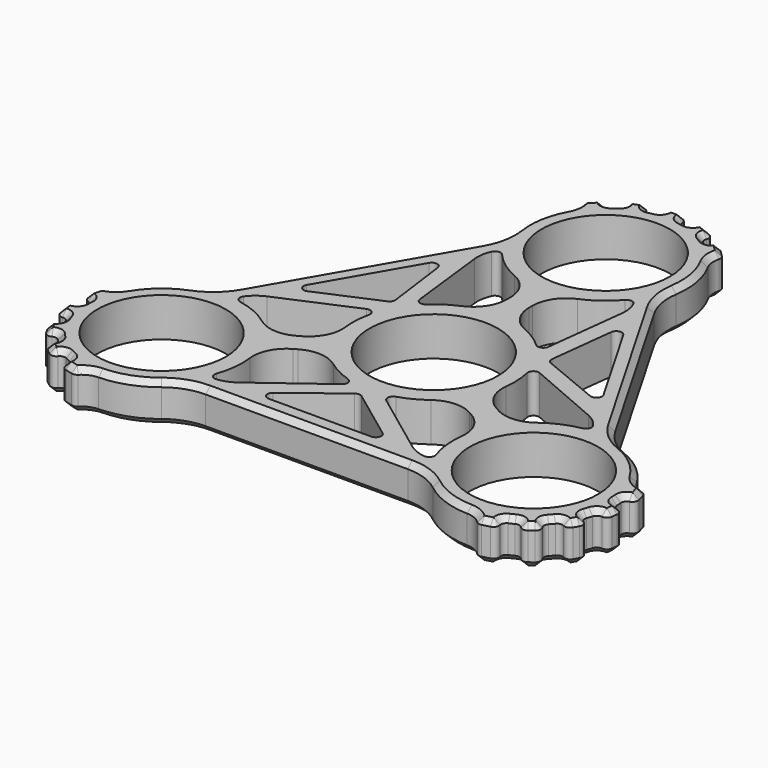
from build123d import *

# Parameters (mm, degrees)
F0_R        = 11.5
F1_DEPTH    = 7
F2_R        = 6
F3_R        = 1
F4_R        = 10
F5_T1_DEPTH = 7
F6_R        = 1
F7_R        = 1
F8_SIZE     = 0.9999


# Not quite as in the source:
# - a fillet or chamfer that OpenCascade refuses, or shapes differently, is made with other operations: its cross-section is extruded or revolved along the edge and cut away or added
# - a fillet or chamfer is up to 0.001 mm smaller than in the source, because OpenCascade refuses the exact size


with BuildPart() as f1:
    # F0 (on Top) → F1 (new body)
    with BuildSketch(Plane.XY):
        with BuildLine():
            Line((-12.5511453661, 48.9298250225), (-11.258699199, 47.6373788554))
            ThreePointArc((-11.258699199, 47.6373788554), (-14.3149781336, 40.8089826842), (-13.5606585567, 33.3659431724))
            Line((-13.5606585567, 33.3659431724), (-35.6760836869, -4.9390967841))
            ThreePointArc((-35.6760836869, -4.9390967841), (-42.4991047739, -8.0073566238), (-46.884529858, -14.0683699078))
            Line((-46.884529858, -14.0683699078), (-48.6500441552, -13.5953017777))
            Line((-48.6500441552, -13.5953017777), (-49.4265012906, -16.4930792565))
            Line((-49.4265012906, -16.4930792565), (-47.6609869933, -16.9661473867))
            ThreePointArc((-47.6609869933, -16.9661473867), (-47.8109324327, -18.3016546262), (-47.8365884719, -19.6453082233))
            Line((-47.8365884719, -19.6453082233), (-49.6487463314, -19.8838833315))
            Line((-49.6487463314, -19.8838833315), (-49.2571677547, -22.8582179156))
            Line((-49.2571677547, -22.8582179156), (-47.4450098953, -22.6196428074))
            ThreePointArc((-47.4450098953, -22.6196428074), (-47.0724649234, -23.9108722469), (-46.5819740425, -25.1620644453))
            Line((-46.5819740425, -25.1620644453), (-48.1648908572, -26.0759618943))
            Line((-48.1648908572, -26.0759618943), (-46.6648908572, -28.6740381057))
            Line((-46.6648908572, -28.6740381057), (-45.0819740425, -27.7601406566))
            ThreePointArc((-45.0819740425, -27.7601406566), (-44.2436552541, -28.810514319), (-43.3116902434, -29.7787624484))
            Line((-43.3116902434, -29.7787624484), (-44.4243812775, -31.2288496362))
            Line((-44.4243812775, -31.2288496362), (-42.0443212567, -33.0551339232))
            Line((-42.0443212567, -33.0551339232), (-40.9316302225, -31.6050467354))
            ThreePointArc((-40.9316302225, -31.6050467354), (-39.7551640539, -32.2546547522), (-38.5236081379, -32.7925518123))
            Line((-38.5236081379, -32.7925518123), (-38.9966762681, -34.5580661095))
            Line((-38.9966762681, -34.5580661095), (-36.0988987892, -35.3345232449))
            Line((-36.0988987892, -35.3345232449), (-35.625830659, -33.5690089476))
            ThreePointArc((-35.625830659, -33.5690089476), (-28.1841266403, -32.8016260604), (-22.1154251302, -28.4268463883))
            Line((-22.1154251302, -28.4268463883), (22.1154251302, -28.4268463883))
            ThreePointArc((22.1154251302, -28.4268463883), (28.1841266403, -32.8016260604), (35.625830659, -33.5690089476))
            Line((35.625830659, -33.5690089476), (36.0988987892, -35.3345232449))
            Line((36.0988987892, -35.3345232449), (38.9966762681, -34.5580661095))
            Line((38.9966762681, -34.5580661095), (38.5236081379, -32.7925518123))
            ThreePointArc((38.5236081379, -32.7925518123), (39.7551640539, -32.2546547522), (40.9316302225, -31.6050467354))
            Line((40.9316302225, -31.6050467354), (42.0443212567, -33.0551339232))
            Line((42.0443212567, -33.0551339232), (44.4243812775, -31.2288496362))
            Line((44.4243812775, -31.2288496362), (43.3116902434, -29.7787624484))
            ThreePointArc((43.3116902434, -29.7787624484), (44.2436552541, -28.810514319), (45.0819740425, -27.7601406566))
            Line((45.0819740425, -27.7601406566), (46.6648908572, -28.6740381057))
            Line((46.6648908572, -28.6740381057), (48.1648908572, -26.0759618943))
            Line((48.1648908572, -26.0759618943), (46.5819740425, -25.1620644453))
            ThreePointArc((46.5819740425, -25.1620644453), (47.0724649234, -23.9108722469), (47.4450098953, -22.6196428074))
            Line((47.4450098953, -22.6196428074), (49.2571677547, -22.8582179156))
            Line((49.2571677547, -22.8582179156), (49.6487463314, -19.8838833315))
            Line((49.6487463314, -19.8838833315), (47.8365884719, -19.6453082233))
            ThreePointArc((47.8365884719, -19.6453082233), (47.8109324327, -18.3016546262), (47.6609869933, -16.9661473867))
            Line((47.6609869933, -16.9661473867), (49.4265012906, -16.4930792565))
            Line((49.4265012906, -16.4930792565), (48.6500441552, -13.5953017777))
            Line((48.6500441552, -13.5953017777), (46.884529858, -14.0683699078))
            ThreePointArc((46.884529858, -14.0683699078), (42.4991047739, -8.0073566238), (35.6760836869, -4.9390967841))
            Line((35.6760836869, -4.9390967841), (13.5606585567, 33.3659431724))
            ThreePointArc((13.5606585567, 33.3659431724), (14.3149781336, 40.8089826842), (11.258699199, 47.6373788554))
            Line((11.258699199, 47.6373788554), (12.5511453661, 48.9298250225))
            Line((12.5511453661, 48.9298250225), (10.4298250225, 51.0511453661))
            Line((10.4298250225, 51.0511453661), (9.1373788554, 49.758699199))
            ThreePointArc((9.1373788554, 49.758699199), (8.0557683788, 50.5563093784), (6.9049582494, 51.2503549587))
            Line((6.9049582494, 51.2503549587), (7.6044250747, 52.9390172548))
            Line((7.6044250747, 52.9390172548), (4.8327864772, 54.0870675519))
            Line((4.8327864772, 54.0870675519), (4.1333196519, 52.3984052558))
            ThreePointArc((4.1333196519, 52.3984052558), (2.8288096692, 52.7213865658), (1.5, 52.9222051019))
            Line((1.5, 52.9222051019), (1.5, 54.75))
            Line((1.5, 54.75), (-1.5, 54.75))
            Line((-1.5, 54.75), (-1.5, 52.9222051019))
            ThreePointArc((-1.5, 52.9222051019), (-2.8288096692, 52.7213865658), (-4.1333196519, 52.3984052558))
            Line((-4.1333196519, 52.3984052558), (-4.8327864772, 54.0870675519))
            Line((-4.8327864772, 54.0870675519), (-7.6044250747, 52.9390172548))
            Line((-7.6044250747, 52.9390172548), (-6.9049582494, 51.2503549587))
            ThreePointArc((-6.9049582494, 51.2503549587), (-8.0557683788, 50.5563093784), (-9.1373788554, 49.758699199))
            Line((-9.1373788554, 49.758699199), (-10.4298250225, 51.0511453661))
            Line((-10.4298250225, 51.0511453661), (-12.5511453661, 48.9298250225))
        make_face()
        with Locations((-33.3419780457, -19.25)):
            Circle(F0_R, mode=Mode.SUBTRACT)
        Polygon((-12.1679823131, -25.4268463883), (-0.1996260557, -16.2213186658), (12.1679823131, -25.4268463883), align=None, mode=Mode.SUBTRACT)
        with BuildLine():
            Line((-19.9046350819, -13.8013474994), (-11.4373429638, -8.9127541157))
            ThreePointArc((-11.4373429638, -8.9127541157), (-7.3686040003, -12.4881413784), (-2.2716589425, -14.3209484899))
            Line((-2.2716589425, -14.3209484899), (-17.1924109007, -25.4268463883))
            Line((-17.1924109007, -25.4268463883), (-20.2234198667, -25.4268463883))
            ThreePointArc((-20.2234198667, -25.4268463883), (-18.8474263976, -19.6474575692), (-19.9046350819, -13.8013474994))
        make_face(mode=Mode.SUBTRACT)
        with BuildLine():
            ThreePointArc((-13.5381346697, 5.193159892), (-14.4993496799, -0.1373275655), (-13.4373429638, -5.4486525006))
            Line((-13.4373429638, -5.4486525006), (-21.9046350819, -10.3372458843))
            ThreePointArc((-21.9046350819, -10.3372458843), (-26.4389105735, -6.4986212717), (-32.1320048438, -4.8005721618))
            Line((-32.1320048438, -4.8005721618), (-30.6165003608, -2.1756413982))
            Line((-30.6165003608, -2.1756413982), (-13.5381346697, 5.193159892))
        make_face(mode=Mode.SUBTRACT)
        with BuildLine():
            ThreePointArc((2.2716589425, -14.3209484899), (7.3686040003, -12.4881413784), (11.4373429638, -8.9127541157))
            Line((11.4373429638, -8.9127541157), (19.9046350819, -13.8013474994))
            ThreePointArc((19.9046350819, -13.8013474994), (18.8474263976, -19.6474575692), (20.2234198667, -25.4268463883))
            Line((20.2234198667, -25.4268463883), (17.1924109007, -25.4268463883))
            Line((17.1924109007, -25.4268463883), (2.2716589425, -14.3209484899))
        make_face(mode=Mode.SUBTRACT)
        with Locations((33.3419780457, -19.25)):
            Circle(F0_R, mode=Mode.SUBTRACT)
        with BuildLine():
            Line((21.9046350819, -10.3372458843), (13.4373429638, -5.4486525006))
            ThreePointArc((13.4373429638, -5.4486525006), (14.4993496799, -0.1373275655), (13.5381346697, 5.193159892))
            Line((13.5381346697, 5.193159892), (30.6165003608, -2.1756413982))
            Line((30.6165003608, -2.1756413982), (32.1320048438, -4.8005721618))
            ThreePointArc((32.1320048438, -4.8005721618), (26.4389105735, -6.4986212717), (21.9046350819, -10.3372458843))
        make_face(mode=Mode.SUBTRACT)
        Circle(F0_R, mode=Mode.SUBTRACT)
        Polygon((-15.9363037538, 23.2512049902), (-13.9482610196, 8.2835405684), (-28.104286067, 2.1756413982), align=None, mode=Mode.SUBTRACT)
        with BuildLine():
            Line((-2, 24.1385933837), (-2, 14.3614066163))
            ThreePointArc((-2, 14.3614066163), (-7.1307456795, 12.6254689439), (-11.2664757273, 9.1277885979))
            Line((-11.2664757273, 9.1277885979), (-13.42408946, 27.6024877865))
            Line((-13.42408946, 27.6024877865), (-11.9085849771, 30.2274185502))
            ThreePointArc((-11.9085849771, 30.2274185502), (-7.5914841759, 26.1460788408), (-2, 24.1385933837))
        make_face(mode=Mode.SUBTRACT)
        with BuildLine():
            ThreePointArc((11.2664757273, 9.1277885979), (7.1307456795, 12.6254689439), (2, 14.3614066163))
            Line((2, 14.3614066163), (2, 24.1385933837))
            ThreePointArc((2, 24.1385933837), (7.5914841759, 26.1460788408), (11.9085849771, 30.2274185502))
            Line((11.9085849771, 30.2274185502), (13.42408946, 27.6024877865))
            Line((13.42408946, 27.6024877865), (11.2664757273, 9.1277885979))
        make_face(mode=Mode.SUBTRACT)
        Polygon((28.104286067, 2.1756413982), (14.1478870753, 7.9377780974), (15.9363037538, 23.2512049902), align=None, mode=Mode.SUBTRACT)
        with Locations((0, 38.5)):
            Circle(F0_R, mode=Mode.SUBTRACT)
    extrude(amount=F1_DEPTH)

    # F2
    f2_edges = [f1.edges().sort_by_distance(p)[0] for p in [
        (-2, 14.361407, 3.5),
        (2, 14.361407, 3.5),
        (2, 24.138593, 3.5),
        (-2, 24.138593, 3.5),
        (-13.437343, -5.448653, 3.5),
        (19.904635, -13.801347, 3.5),
        (-19.904635, -13.801347, 3.5),
        (-11.437343, -8.912754, 3.5),
        (-21.904635, -10.337246, 3.5),
        (21.904635, -10.337246, 3.5),
        (11.437343, -8.912754, 3.5),
        (13.437343, -5.448653, 3.5),
        (-30.6165, -2.175641, 3.5),
        (-17.192411, -25.426846, 3.5),
        (17.192411, -25.426846, 3.5),
        (13.424089, 27.602488, 3.5),
        (30.6165, -2.175641, 3.5),
        (-13.424089, 27.602488, 3.5),
    ]]
    fillet(f2_edges, radius=F2_R)

    # F3
    f3_edges = [f1.edges().sort_by_distance(p)[0] for p in [
        (-11.266476, 9.127789, 3.5),
        (-13.538135, 5.19316, 3.5),
        (-2.271659, -14.320948, 3.5),
        (2.271659, -14.320948, 3.5),
        (13.538135, 5.19316, 3.5),
        (11.266476, 9.127789, 3.5),
        (32.132005, -4.800572, 3.5),
        (20.22342, -25.426846, 3.5),
        (-20.22342, -25.426846, 3.5),
        (-32.132005, -4.800572, 3.5),
        (11.908585, 30.227419, 3.5),
        (-11.908585, 30.227419, 3.5),
        (-15.936304, 23.251205, 3.5),
        (-28.104286, 2.175641, 3.5),
        (28.104286, 2.175641, 3.5),
        (15.936304, 23.251205, 3.5),
        (12.167982, -25.426846, 3.5),
        (-12.167982, -25.426846, 3.5),
        (-13.948261, 8.283541, 3.5),
        (-0.199626, -16.221319, 3.5),
        (14.147887, 7.937778, 3.5),
    ]]
    fillet(f3_edges, radius=F3_R)

    # F4
    f4_edges = [f1.edges().sort_by_distance(p)[0] for p in [
        (-13.560659, 33.365943, 3.5),
        (13.560659, 33.365943, 3.5),
        (-35.676084, -4.939097, 3.5),
        (-22.115425, -28.426846, 3.5),
        (22.115425, -28.426846, 3.5),
        (35.676084, -4.939097, 3.5),
    ]]
    fillet(f4_edges, radius=F4_R)

    # F5: fillet of radius 4 on 6 edges, made by hand

    # F5_s2 → F5_t1 (join)
    with BuildSketch(Plane.XY):
        with BuildLine():
            ThreePointArc((-12.5511453661, 48.9298250225), (-12.2396379947, 47.1713300782), (-12.7244772243, 45.4525304292))
            ThreePointArc((-12.7244772243, 45.4525304292), (-12.0412448899, 46.5782684717), (-11.258699199, 47.6373788554))
            Line((-11.258699199, 47.6373788554), (-12.5511453661, 48.9298250225))
        make_face()
        with BuildLine():
            ThreePointArc((12.7244772243, 45.4525304292), (12.2396379947, 47.1713300782), (12.5511453661, 48.9298250225))
            Line((12.5511453661, 48.9298250225), (11.258699199, 47.6373788554))
            ThreePointArc((11.258699199, 47.6373788554), (12.0412448899, 46.5782684717), (12.7244772243, 45.4525304292))
        make_face()
        with BuildLine():
            ThreePointArc((-45.7252846301, -11.7065446885), (-46.9713891754, -12.9858276025), (-48.6500441552, -13.5953017777))
            Line((-48.6500441552, -13.5953017777), (-46.884529858, -14.0683699078))
            ThreePointArc((-46.884529858, -14.0683699078), (-46.3585862058, -12.861110268), (-45.7252846301, -11.7065446885))
        make_face()
        with BuildLine():
            ThreePointArc((-33.0008074058, -33.7459857407), (-34.7317511806, -34.1855024756), (-36.0988987892, -35.3345232449))
            Line((-36.0988987892, -35.3345232449), (-35.625830659, -33.5690089476))
            ThreePointArc((-35.625830659, -33.5690089476), (-34.3173413159, -33.7171582037), (-33.0008074058, -33.7459857407))
        make_face()
        with BuildLine():
            ThreePointArc((36.0988987892, -35.3345232449), (34.7317511806, -34.1855024756), (33.0008074058, -33.7459857407))
            ThreePointArc((33.0008074058, -33.7459857407), (34.3173413159, -33.7171582037), (35.625830659, -33.5690089476))
            Line((35.625830659, -33.5690089476), (36.0988987892, -35.3345232449))
        make_face()
        with BuildLine():
            ThreePointArc((45.7252846301, -11.7065446885), (46.9713891754, -12.9858276025), (48.6500441552, -13.5953017777))
            Line((48.6500441552, -13.5953017777), (46.884529858, -14.0683699078))
            ThreePointArc((46.884529858, -14.0683699078), (46.3585862058, -12.861110268), (45.7252846301, -11.7065446885))
        make_face()
    extrude(amount=F5_T1_DEPTH)

    # F6
    f6_edges = [f1.edges().sort_by_distance(p)[0] for p in [
        (-9.137379, 49.758699, 3.5),
        (-6.904958, 51.250355, 3.5),
        (-4.13332, 52.398405, 3.5),
        (-1.5, 52.922205, 3.5),
        (1.5, 52.922205, 3.5),
        (6.904958, 51.250355, 3.5),
        (4.13332, 52.398405, 3.5),
        (9.137379, 49.758699, 3.5),
        (-47.660987, -16.966147, 3.5),
        (-47.44501, -22.619643, 3.5),
        (-40.93163, -31.605047, 3.5),
        (-45.081974, -27.760141, 3.5),
        (-47.836588, -19.645308, 3.5),
        (-46.581974, -25.162064, 3.5),
        (-43.31169, -29.778762, 3.5),
        (-38.523608, -32.792552, 3.5),
        (47.660987, -16.966147, 3.5),
        (47.44501, -22.619643, 3.5),
        (45.081974, -27.760141, 3.5),
        (40.93163, -31.605047, 3.5),
        (38.523608, -32.792552, 3.5),
        (43.31169, -29.778762, 3.5),
        (46.581974, -25.162064, 3.5),
        (47.836588, -19.645308, 3.5),
    ]]
    fillet(f6_edges, radius=F6_R)

    # F7
    f7_edges = [f1.edges().sort_by_distance(p)[0] for p in [
        (-7.604425, 52.939017, 3.5),
        (-4.832786, 54.087068, 3.5),
        (-12.551145, 48.929825, 3.5),
        (-10.429825, 51.051145, 3.5),
        (-1.5, 54.75, 3.5),
        (1.5, 54.75, 3.5),
        (4.832786, 54.087068, 3.5),
        (7.604425, 52.939017, 3.5),
        (10.429825, 51.051145, 3.5),
        (12.551145, 48.929825, 3.5),
        (-48.650044, -13.595302, 3.5),
        (-49.426501, -16.493079, 3.5),
        (-49.648746, -19.883883, 3.5),
        (-49.257168, -22.858218, 3.5),
        (-48.164891, -26.075962, 3.5),
        (-46.664891, -28.674038, 3.5),
        (-44.424381, -31.22885, 3.5),
        (-42.044321, -33.055134, 3.5),
        (-38.996676, -34.558066, 3.5),
        (-36.098899, -35.334523, 3.5),
        (36.098899, -35.334523, 3.5),
        (38.996676, -34.558066, 3.5),
        (42.044321, -33.055134, 3.5),
        (44.424381, -31.22885, 3.5),
        (46.664891, -28.674038, 3.5),
        (48.164891, -26.075962, 3.5),
        (49.257168, -22.858218, 3.5),
        (49.648746, -19.883883, 3.5),
        (49.426501, -16.493079, 3.5),
        (48.650044, -13.595302, 3.5),
    ]]
    fillet(f7_edges, radius=F7_R)

    # F8 (size 1 in the source; OpenCascade refuses exactly that, so slightly less here)
    f8_edges = [f1.edges().sort_by_distance(p)[0] for p in [
        (0, -28.426846, 7),
        (0, -28.426846, 0),
        (9.118065, 50.086816, 0),
        (10.441199, 50.637254, 0),
        (8.055768, 50.556309, 0),
        (11.624046, 49.856924, 0),
        (7.21549, 51.358076, 0),
        (12.370311, 48.921356, 0),
        (7.217687, 52.791136, 0),
        (12.263141, 46.894133, 0),
        (6.218606, 53.513042, 0),
        (14.27612, 41.038187, 0),
        (5.001684, 53.709035, 0),
        (14.407264, 33.017162, 0),
        (3.989911, 52.694155, 0),
        (24.618371, 14.213423, 0),
        (2.82881, 52.721387, 0),
        (35.797333, -4.031524, 0),
        (1.745671, 53.140562, 0),
        (42.678173, -8.155611, 0),
        (1.199292, 54.465377, 0),
        (46.743081, -12.826875, 0),
        (0, 54.75, 0),
        (48.552292, -13.747674, 0),
        (-1.199292, 54.465377, 0),
        (48.989386, -14.861743, 0),
        (-1.745671, 53.140562, 0),
        (49.073748, -16.276284, 0),
        (-2.82881, 52.721387, 0),
        (47.935488, -17.146932, 0),
        (-3.989911, 52.694155, 0),
        (47.810932, -18.301655, 0),
        (-5.001684, 53.709035, 0),
        (48.085144, -19.43024, 0),
        (-6.218606, 53.513042, 0),
        (49.327308, -20.144868, 0),
        (-7.217687, 52.791136, 0),
        (49.452957, -21.371051, 0),
        (-7.21549, 51.358076, 0),
        (49.01423, -22.522932, 0),
        (-8.055768, 50.556309, 0),
        (47.629432, -22.891713, 0),
        (-9.118065, 50.086816, 0),
        (47.072465, -23.910872, 0),
        (-10.441199, 50.637254, 0),
        (46.893912, -25.058486, 0),
        (-11.624046, 49.856924, 0),
        (47.768046, -26.194071, 0),
        (-12.370311, 48.921356, 0),
        (47.414891, -27.375, 0),
        (-12.263141, 46.894133, 0),
        (46.568754, -28.271306, 0),
        (-14.27612, 41.038187, 0),
        (45.148241, -28.082076, 0),
        (-14.407264, 33.017162, 0),
        (44.243655, -28.810514, 0),
        (-24.618371, 14.213423, 0),
        (43.639521, -29.802442, 0),
        (-35.797333, -4.031524, 0),
        (44.012546, -31.186103, 0),
        (-42.678173, -8.155611, 0),
        (43.234351, -32.141992, 0),
        (-46.743081, -12.826875, 0),
        (42.109622, -32.646268, 0),
        (-48.552292, -13.747674, 0),
        (40.869654, -31.927836, 0),
        (-48.989386, -14.861743, 0),
        (39.755164, -32.254655, 0),
        (-49.073748, -16.276284, 0),
        (38.817423, -32.939884, 0),
        (-47.935488, -17.146932, 0),
        (38.632549, -34.360971, 0),
        (-47.810932, -18.301655, 0),
        (37.36534, -34.995181, 0),
        (-48.085144, -19.43024, 0),
        (36.181982, -35.173681, 0),
        (-49.327308, -20.144868, 0),
        (34.47994, -34.067258, 0),
        (-49.452957, -21.371051, 0),
        (28.402053, -32.882576, 0),
        (-49.01423, -22.522932, 0),
        (21.390069, -28.985638, 0),
        (-47.629432, -22.891713, 0),
        (-47.072465, -23.910872, 0),
        (-21.390069, -28.985638, 0),
        (-46.893912, -25.058486, 0),
        (-28.402053, -32.882576, 0),
        (-47.768046, -26.194071, 0),
        (-34.47994, -34.067258, 0),
        (-47.414891, -27.375, 0),
        (-36.181982, -35.173681, 0),
        (-46.568754, -28.271306, 0),
        (-37.36534, -34.995181, 0),
        (-45.148241, -28.082076, 0),
        (-38.632549, -34.360971, 0),
        (-44.243655, -28.810514, 0),
        (-38.817423, -32.939884, 0),
        (-43.639521, -29.802442, 0),
        (-39.755164, -32.254655, 0),
        (-44.012546, -31.186103, 0),
        (-40.869654, -31.927836, 0),
        (-43.234351, -32.141992, 0),
        (-42.109622, -32.646268, 0),
        (9.118065, 50.086816, 7),
        (10.441199, 50.637254, 7),
        (8.055768, 50.556309, 7),
        (11.624046, 49.856924, 7),
        (7.21549, 51.358076, 7),
        (12.370311, 48.921356, 7),
        (7.217687, 52.791136, 7),
        (12.263141, 46.894133, 7),
        (6.218606, 53.513042, 7),
        (14.27612, 41.038187, 7),
        (5.001684, 53.709035, 7),
        (14.407264, 33.017162, 7),
        (3.989911, 52.694155, 7),
        (24.618371, 14.213423, 7),
        (2.82881, 52.721387, 7),
        (35.797333, -4.031524, 7),
        (1.745671, 53.140562, 7),
        (42.678173, -8.155611, 7),
        (1.199292, 54.465377, 7),
        (46.743081, -12.826875, 7),
        (0, 54.75, 7),
        (48.552292, -13.747674, 7),
        (-1.199292, 54.465377, 7),
        (48.989386, -14.861743, 7),
        (-1.745671, 53.140562, 7),
        (49.073748, -16.276284, 7),
        (-2.82881, 52.721387, 7),
        (47.935488, -17.146932, 7),
        (-3.989911, 52.694155, 7),
        (47.810932, -18.301655, 7),
        (-5.001684, 53.709035, 7),
        (48.085144, -19.43024, 7),
        (-6.218606, 53.513042, 7),
        (49.327308, -20.144868, 7),
        (-7.217687, 52.791136, 7),
        (49.452957, -21.371051, 7),
        (-7.21549, 51.358076, 7),
        (49.01423, -22.522932, 7),
        (-8.055768, 50.556309, 7),
        (47.629432, -22.891713, 7),
        (-9.118065, 50.086816, 7),
        (47.072465, -23.910872, 7),
        (-10.441199, 50.637254, 7),
        (46.893912, -25.058486, 7),
        (-11.624046, 49.856924, 7),
        (47.768046, -26.194071, 7),
        (-12.370311, 48.921356, 7),
        (47.414891, -27.375, 7),
        (-12.263141, 46.894133, 7),
        (46.568754, -28.271306, 7),
        (-14.27612, 41.038187, 7),
        (45.148241, -28.082076, 7),
        (-14.407264, 33.017162, 7),
        (44.243655, -28.810514, 7),
        (-24.618371, 14.213423, 7),
        (43.639521, -29.802442, 7),
        (-35.797333, -4.031524, 7),
        (44.012546, -31.186103, 7),
        (-42.678173, -8.155611, 7),
        (43.234351, -32.141992, 7),
        (-46.743081, -12.826875, 7),
        (42.109622, -32.646268, 7),
        (-48.552292, -13.747674, 7),
        (40.869654, -31.927836, 7),
        (-48.989386, -14.861743, 7),
        (39.755164, -32.254655, 7),
        (-49.073748, -16.276284, 7),
        (38.817423, -32.939884, 7),
        (-47.935488, -17.146932, 7),
        (38.632549, -34.360971, 7),
        (-47.810932, -18.301655, 7),
        (37.36534, -34.995181, 7),
        (-48.085144, -19.43024, 7),
        (36.181982, -35.173681, 7),
        (-49.327308, -20.144868, 7),
        (34.47994, -34.067258, 7),
        (-49.452957, -21.371051, 7),
        (28.402053, -32.882576, 7),
        (-49.01423, -22.522932, 7),
        (21.390069, -28.985638, 7),
        (-47.629432, -22.891713, 7),
        (-47.072465, -23.910872, 7),
        (-21.390069, -28.985638, 7),
        (-46.893912, -25.058486, 7),
        (-28.402053, -32.882576, 7),
        (-47.768046, -26.194071, 7),
        (-34.47994, -34.067258, 7),
        (-47.414891, -27.375, 7),
        (-36.181982, -35.173681, 7),
        (-46.568754, -28.271306, 7),
        (-37.36534, -34.995181, 7),
        (-45.148241, -28.082076, 7),
        (-38.632549, -34.360971, 7),
        (-44.243655, -28.810514, 7),
        (-38.817423, -32.939884, 7),
        (-43.639521, -29.802442, 7),
        (-39.755164, -32.254655, 7),
        (-44.012546, -31.186103, 7),
        (-40.869654, -31.927836, 7),
        (-43.234351, -32.141992, 7),
        (-42.109622, -32.646268, 7),
    ]]
    chamfer(f8_edges, length=F8_SIZE)


solid = f1.part
